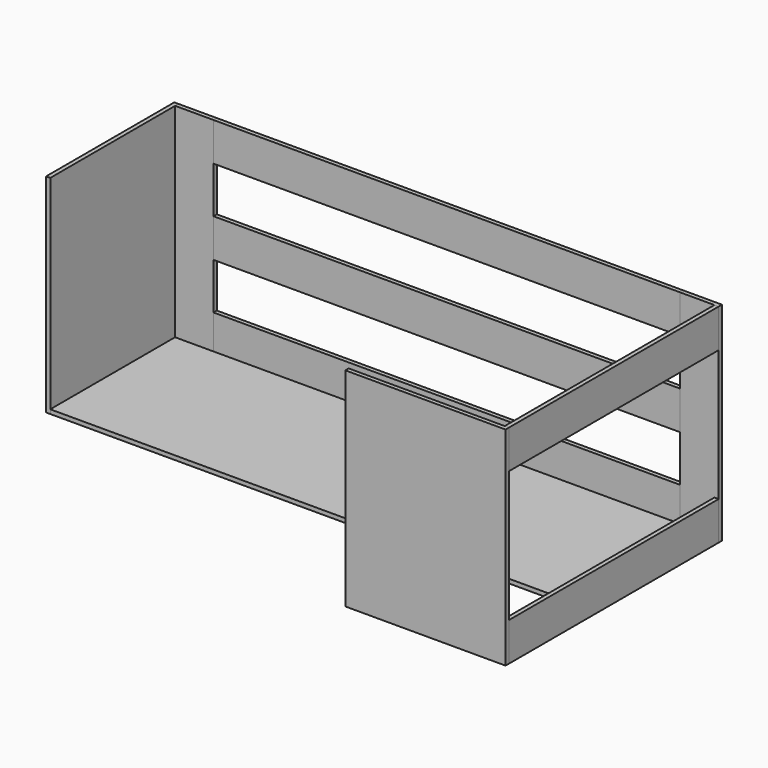
from build123d import *

# Parameters (mm, degrees)
F2_DEPTH  = 15.875
F1_W      = 1774.825
F1_H      = 146.05
F3_DEPTH  = 15.875
F4_DEPTH  = 15.875
F5_DEPTH  = 15.875
F6_DEPTH  = 15.875
F7_W      = 609.6
F7_H      = 790.575
F8_DEPTH  = 15.875
F9_W      = 15.875
F9_H      = 146.05
F10_DEPTH = 996.95
F11_W     = 609.6
F11_H     = 790.575
F12_DEPTH = 15.875
F13_W     = 2050.8346557617
F13_H     = 593.2907479912
F14_DEPTH = 15.875


# Not quite as in the source:
# - a variable given as a bare number and used for a length is read in inches; the dataset says mm whatever the document's units were


with BuildPart() as f2:
    # F1 (on Front) → F2 (new body)
    with BuildSketch(Plane.XZ):
        Polygon((0, 812.0033606444), (0, 21.4283606444), (146.05, 21.4283606444), (146.05, 167.4783606444), (146.05, 343.6908606444), (146.05, 489.7408606444), (146.05, 665.9533606444), (146.05, 812.0033606444), align=None)
    extrude(amount=F2_DEPTH)


with BuildPart() as f3:
    # F1 (on Front) → F3 (new body)
    with BuildSketch(Plane.XZ):
        with Locations((1033.4625, 738.9783606444)):
            Rectangle(F1_W, F1_H)
    extrude(amount=F3_DEPTH)


with BuildPart() as f4:
    # F1 (on Front) → F4 (new body)
    with BuildSketch(Plane.XZ):
        with Locations((1033.4625, 416.7158606444)):
            Rectangle(F1_W, F1_H)
    extrude(amount=F4_DEPTH)


with BuildPart() as f5:
    # F1 (on Front) → F5 (new body)
    with BuildSketch(Plane.XZ):
        with Locations((1033.4625, 94.4533606444)):
            Rectangle(F1_W, F1_H)
    extrude(amount=F5_DEPTH)


with BuildPart() as f6:
    # F1 (on Front) → F6 (new body)
    with BuildSketch(Plane.XZ):
        Polygon((1920.875, 167.4783606444), (1920.875, 21.4283606444), (2066.925, 21.4283606444), (2066.925, 812.0033606444), (1920.875, 812.0033606444), (1920.875, 665.9533606444), (1920.875, 489.7408606444), (1920.875, 343.6908606444), align=None)
    extrude(amount=F6_DEPTH)


with BuildPart() as f8:
    # F7 (on face) → F8 (new body)
    with BuildSketch(Plane(origin=(0, 0, 0), x_dir=(0, -1, 0), z_dir=(-1, 0, 0))):
        with Locations((304.8, 416.7158606444)):
            Rectangle(F7_W, F7_H)
    extrude(amount=F8_DEPTH)


with BuildPart() as f10:
    # F9 (on face) → F10 (new body)
    with BuildSketch(Plane.XZ.offset(15.875)):
        with Locations((2058.9875, 738.9783606444)):
            Rectangle(F9_W, F9_H)
    extrude(amount=F10_DEPTH)


with BuildPart() as f10b:
    # F9 (on face) → F10, piece 2 (new body)
    with BuildSketch(Plane.XZ.offset(15.875)):
        with Locations((2058.9875, 94.4533606444)):
            Rectangle(F9_W, F9_H)
    extrude(amount=F10_DEPTH)


with BuildPart() as f12:
    # F11 (on face) → F12 (new body)
    with BuildSketch(Plane.XZ.offset(1012.825)):
        with Locations((1762.125, 416.7158606444)):
            Rectangle(F11_W, F11_H)
    extrude(amount=F12_DEPTH)


with BuildPart() as f14:
    # F13 (on face) → F14 (new body)
    with BuildSketch(Plane(origin=(0, 0, 21.4283606444), x_dir=(1, 0, 0), z_dir=(0, 0, -1))):
        with Locations((1025.4173278809, 312.9546260044)):
            Rectangle(F13_W, F13_H)
    extrude(amount=-F14_DEPTH)


solid = Compound([f2.part, f3.part, f4.part, f5.part, f6.part, f8.part, f10.part, f10b.part, f12.part, f14.part])
